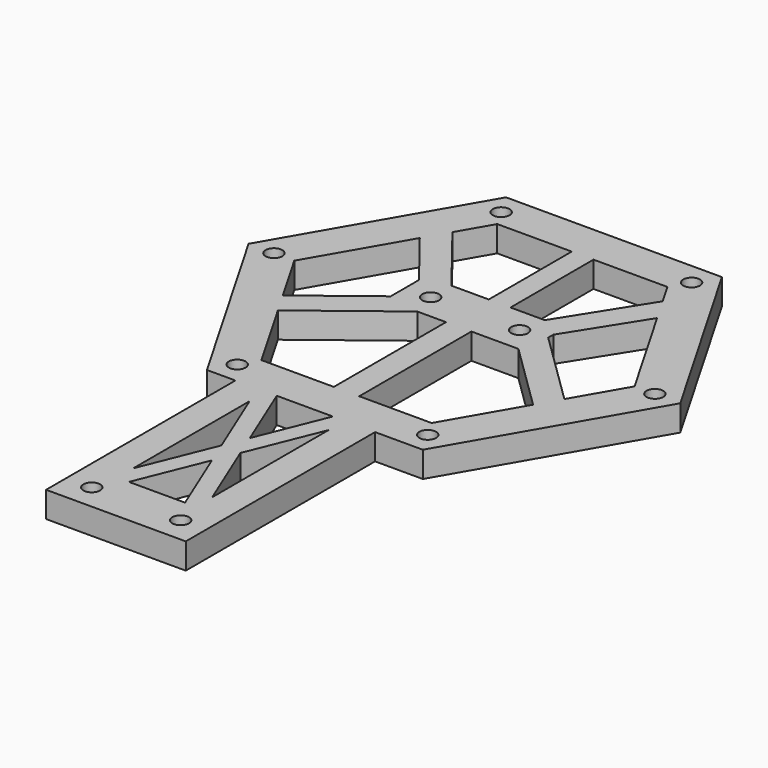
from build123d import *

# Parameters (mm, degrees)
F0_R     = 1.65
F0_W     = 4.2823543772
F0_H     = 20.4163840114
F0_W_2   = 5
F0_H_2   = 27.6073180421
F1_DEPTH = 5.08


# Not quite as in the source:
# - a feature names something its author has since deleted; it is built from what else it names


with BuildPart() as f1:
    # F0 (on Top) → F1 (new body)
    with BuildSketch(Plane.XY):
        Polygon((21.25, 36.8060796608), (-21.25, 36.8060796608), (-42.5, 0), (-21.25, -36.8060796608), (-15.6452442706, -36.8060796608), (-9.6452442706, -36.8060796608), (-7.5036888061, -36.8060796608), (3.5473197586, -36.8060796608), (5.8547557294, -36.8060796608), (11.8547557294, -36.8060796608), (21.25, -36.8060796608), (42.5, 0), align=None)
        with Locations((-18.75, -32.4759526419)):
            Circle(F0_R, mode=Mode.SUBTRACT)
        with Locations((18.75, -32.4759526419)):
            Circle(F0_R, mode=Mode.SUBTRACT)
        with Locations((-37.5, 0)):
            Circle(F0_R, mode=Mode.SUBTRACT)
        with Locations((-18.75, 32.4759526419)):
            Circle(F0_R, mode=Mode.SUBTRACT)
        Polygon((-20.4496354018, 22.6038945413), (-16.75, 29.0118510268), (-2.0811383147, 29.0118510268), (2.2012160625, 29.0118510268), (16.75, 29.0118510268), (19.1722516141, 24.8163881624), (21.9975489559, 19.92282962), (33.5, 0), (27.7061208369, -10.0352930835), (25.125, -14.5059255134), (16.75, -29.0118510268), (2.497308068, -29.0118510268), (-2.502691932, -29.0118510268), (-16.75, -29.0118510268), (-25.125, -14.5059255134), (-27.6475357555, -10.1367654209), (-33.5, 0), (-23.1427541029, 17.9392761202), align=None, mode=Mode.SUBTRACT)
        with Locations((37.5, 0)):
            Circle(F0_R, mode=Mode.SUBTRACT)
        with Locations((18.75, 32.4759526419)):
            Circle(F0_R, mode=Mode.SUBTRACT)
        Polygon((2.2012160625, 8.5954670154), (-2.0811383147, 8.5954670154), (-9.4379286368, 8.5954670154), (-14.5152442706, 8.5954670154), (-14.5152442706, 6.9638797721), (-14.5152442706, 0), (-14.5152442706, -1.4045329846), (-8.1520013755, -1.4045329846), (-2.502691932, -1.4045329846), (2.497308068, -1.4045329846), (11.7475565604, -1.4045329846), (12.9847557294, -1.4045329846), (12.9847557294, 4.3822885496), (12.9847557294, 5.62991663), (12.9847557294, 8.5954670154), (8.9436992999, 8.5954670154), align=None)
        with Locations((-9.5152442706, 3.5954670154)):
            Circle(F0_R, mode=Mode.SUBTRACT)
        with Locations((7.9847557294, 3.5954670154)):
            Circle(F0_R, mode=Mode.SUBTRACT)
        Polygon((-9.6452442706, -36.8060796608), (-15.6452442706, -36.8060796608), (-15.6452442706, -73.3945329846), (-9.6452442706, -73.3945329846), (-9.6452442706, -69.4588214522), (-9.6452442706, -40.8093024077), align=None)
        Polygon((11.8547557294, -73.3945329846), (11.8547557294, -36.8060796608), (5.8547557294, -36.8060796608), (5.8547557294, -40.7417911932), (5.8547557294, -69.3913102377), (5.8547557294, -73.3945329846), align=None)
        Polygon((5.8547557294, -40.7417911932), (5.8547557294, -36.8060796608), (3.5473197586, -36.8060796608), (-1.9379455123, -50.3825876202), (0.0250296589, -55.1708695493), align=None)
        Polygon((-7.5036888061, -36.8060796608), (-9.6452442706, -36.8060796608), (-9.6452442706, -40.8093024077), (-3.8155182001, -55.0297430961), (-1.9379455123, -50.3825876202), align=None)
        Polygon((0.0250296589, -55.1708695493), (-1.9379455123, -50.3825876202), (-3.8155182001, -55.0297430961), (-1.8525430289, -59.8180250252), align=None)
        Polygon((-9.6452442706, -69.4588214522), (-9.6452442706, -73.3945329846), (-7.3378082997, -73.3945329846), (-1.8525430289, -59.8180250252), (-3.8155182001, -55.0297430961), align=None)
        Polygon((3.713200265, -73.3945329846), (5.8547557294, -73.3945329846), (5.8547557294, -69.3913102377), (0.0250296589, -55.1708695493), (-1.8525430289, -59.8180250252), align=None)
        Polygon((-9.6452442706, -73.3945329846), (-15.6452442706, -73.3945329846), (-15.6452442706, -83.3945329846), (11.8547557294, -83.3945329846), (11.8547557294, -73.3945329846), (5.8547557294, -73.3945329846), (3.713200265, -73.3945329846), (-7.3378082997, -73.3945329846), align=None)
        with Locations((-10.6452442706, -78.3945329846)):
            Circle(F0_R, mode=Mode.SUBTRACT)
        with Locations((6.8547557294, -78.3945329846)):
            Circle(F0_R, mode=Mode.SUBTRACT)
        Polygon((-9.4379286368, 8.5954670154), (-20.4496354018, 22.6038945413), (-23.1427541029, 17.9392761202), (-14.5152442706, 6.9638797721), (-14.5152442706, 8.5954670154), align=None)
        with Locations((0.0600388739, 18.8036590211)):
            Rectangle(F0_W, F0_H)
        Polygon((21.9975489559, 19.92282962), (19.1722516141, 24.8163881624), (8.9436992999, 8.5954670154), (12.9847557294, 8.5954670154), (12.9847557294, 5.62991663), align=None)
        Polygon((25.125, -14.5059255134), (27.7061208369, -10.0352930835), (12.9847557294, 4.3822885496), (12.9847557294, -1.4045329846), (11.7475565604, -1.4045329846), align=None)
        Polygon((-14.5152442706, 0), (-27.6475357555, -10.1367654209), (-25.125, -14.5059255134), (-8.1520013755, -1.4045329846), (-14.5152442706, -1.4045329846), align=None)
        with Locations((-0.002691932, -15.2081920057)):
            Rectangle(F0_W_2, F0_H_2)
    extrude(amount=F1_DEPTH)


solid = f1.part
